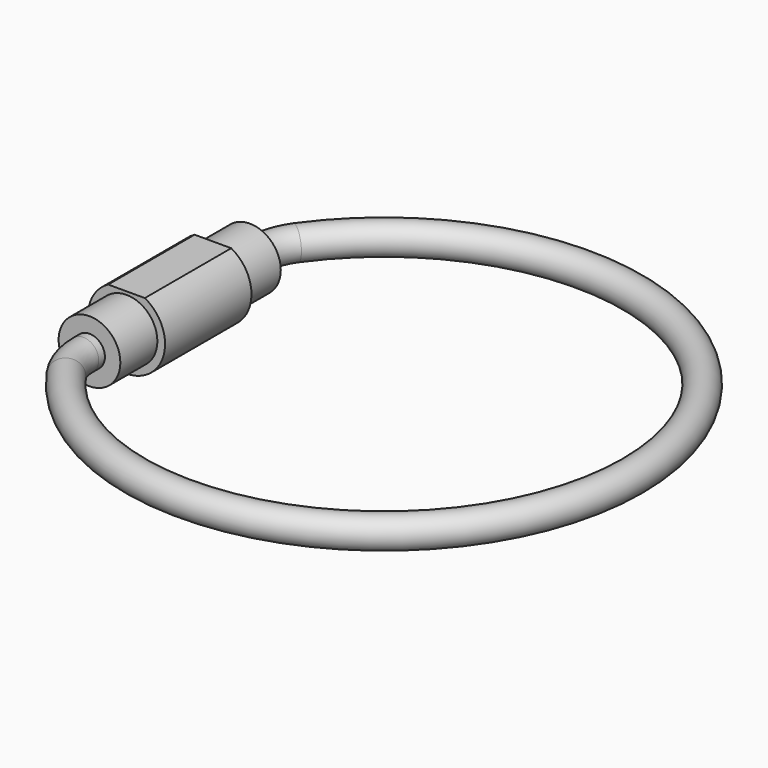
from build123d import *

# Parameters (mm, degrees)
F0_R     = 2.5
F1_DEPTH = 3.5
F2_W     = 2.3748684174
F2_H     = 0.3
F3_DEPTH = 7.001
F4_R     = 2
F5_DEPTH = 3
F7_R     = 1


# Not quite as in the source:
# - a pattern or mirror of a feature is missing from the dataset's text; its kind, count and spacing are read off the source's solid


with BuildPart() as f1:
    # F0 (on Front) → F1 (new body, symmetric)
    with BuildSketch(Plane.XZ):
        Circle(F0_R)
    extrude(amount=F1_DEPTH, both=True)

    # F2 (on face) → F3 (cut, through all)
    with BuildSketch(Plane.XZ.offset(3.5)):
        with Locations((0, 2.35)):
            Rectangle(F2_W, F2_H)
    extrude(amount=-F3_DEPTH, mode=Mode.SUBTRACT)

    # F4 (on face) → F5 (join)
    with BuildSketch(Plane.XZ.offset(3.5)):
        Circle(F4_R)
    f5 = extrude(amount=F5_DEPTH)

    # F5_copies: F5 across plane
    add(f5.mirror(Plane.ZX))

    # F8: sweep along a path in F6
    with BuildLine(Plane.XY) as f8_path:
        Line((0, 7), (0, -7))
        ThreePointArc((0, -7), (0.1882968799, -8.2128146291), (0.7354596623, -9.3114446529))
        ThreePointArc((0.7354596623, -9.3114446529), (30, 0), (0.7354596623, 9.3114446529))
        ThreePointArc((0.7354596623, 9.3114446529), (0.1882968799, 8.2128146291), (0, 7))
    # F7 (on face) → F8 (sweep)
    with BuildSketch(Plane.XZ.offset(6.5)):
        Circle(F7_R)
    sweep(path=f8_path.line)


solid = f1.part
